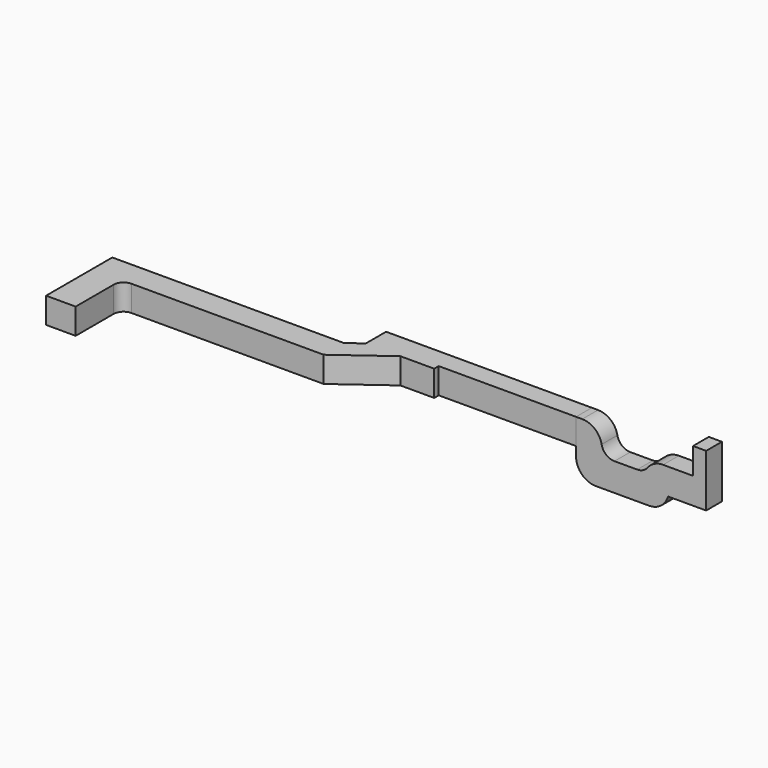
from build123d import *

# Parameters (mm, degrees)
F0_W        = 4.5
F0_H        = 8.74
F0_W_2      = 20.9
F0_H_2      = 3
F1_DEPTH    = 3.92
F0_W_3      = 19.8
F2_DEPTH    = 8.3
F3_DEPTH    = 1.88
F4_W        = 5.8
F4_H        = 2.18
F5_DEPTH    = 25
F6_T1_DEPTH = 18
F6_T3_DEPTH = 17.4287906631
F6_T5_DEPTH = 16.9987425023
F7_R        = 2
F8_R        = 1.5


# Not quite as in the source:
# - a fillet or chamfer that OpenCascade refuses, or shapes differently, is made with other operations: its cross-section is extruded or revolved along the edge and cut away or added
# - a feature names something its author has since deleted; it is built from what else it names


with BuildPart() as f1:
    # F0 (on Top) → F1 (new body)
    with BuildSketch(Plane.XY):
        with Locations((2.25, 4.37)):
            Rectangle(F0_W, F0_H)
        Polygon((0, 12.6), (0, 8.74), (4.5, 8.74), (35.25, 8.74), (35.25, 12.6), align=None)
        Polygon((35.25, 12.6), (35.25, 8.74), (42.6136363636, 14.14), (37.35, 14.14), align=None)
        Polygon((37.35, 14.14), (42.6136363636, 14.14), (47.76, 14.14), (47.76, 15), (47.76, 18), (37.35, 18), align=None)
        with Locations((58.21, 16.5)):
            Rectangle(F0_W_2, F0_H_2)
    extrude(amount=-F1_DEPTH)

    # F8
    f8_edges = [f1.edges().sort_by_distance(p)[0] for p in [
        (4.5, 8.74, -1.96),
    ]]
    fillet(f8_edges, radius=F8_R)


with BuildPart() as f2:
    # F0 (on Top) → F2 (new body)
    with BuildSketch(Plane.XY):
        with Locations((78.56, 16.5)):
            Rectangle(F0_W_3, F0_H_2)
    extrude(amount=-F2_DEPTH)

    # F0 (on Top) → F3 (join)
    with BuildSketch(Plane.XY):
        with Locations((78.56, 16.5)):
            Rectangle(F0_W_3, F0_H_2)
    extrude(amount=F3_DEPTH)

    # F4 (on face) → F5 (cut)
    with BuildSketch(Plane(origin=(0, 18, 0), x_dir=(-1, 0, 0), z_dir=(0, 1, 0))):
        with Locations((-85.56, -7.21)):
            Rectangle(F4_W, F4_H)
        Polygon((-68.66, 1.88), (-86.46, 1.88), (-86.46, -2.12), (-82.66, -2.12), (-79.1077613831, -2.12), (-79.1077613831, -4.0423134342), (-72.6052895188, -4.0423134342), (-72.6052895188, 0), (-68.66, 0), align=None)
    extrude(amount=-F5_DEPTH, mode=Mode.SUBTRACT)

    # F6: fillet of radius 3 on 4 edges, made by hand

    # F6_s2 → F6_t1 (cut)
    with BuildSketch(Plane.XZ.offset(-25.5)):
        with BuildLine():
            ThreePointArc((68.66, -5.3), (69.5386796564, -7.4213203436), (71.66, -8.3))
            Line((71.66, -8.3), (68.66, -8.3))
            Line((68.66, -8.3), (68.66, -5.3))
        make_face()
        with BuildLine():
            ThreePointArc((69.6052895188, 0), (71.7266098624, -0.8786796564), (72.6052895188, -3))
            Line((72.6052895188, -3), (72.6052895188, 0))
            Line((72.6052895188, 0), (69.6052895188, 0))
        make_face()
    extrude(amount=F6_T1_DEPTH, mode=Mode.SUBTRACT)

    # F6_s4 → F6_t3 (cut)
    with BuildSketch(Plane.XZ.offset(-25.2143953316)):
        with BuildLine():
            ThreePointArc((79.7742418674, -8.3), (81.5825559994, -7.6937418407), (82.66, -6.12))
            Line((82.66, -6.12), (82.66, -8.3))
            Line((82.66, -8.3), (79.7742418674, -8.3))
        make_face()
    extrude(amount=F6_T3_DEPTH, mode=Mode.SUBTRACT)

    # F6_s6 → F6_t5 (cut)
    with BuildSketch(Plane.XZ.offset(-24.9993712512)):
        with BuildLine():
            ThreePointArc((81.9075098835, -2.12), (80.2094315133, -2.6468380868), (79.1077613831, -4.0423134342))
            Line((79.1077613831, -4.0423134342), (79.1077613831, -2.12))
            Line((79.1077613831, -2.12), (81.9075098835, -2.12))
        make_face()
    extrude(amount=F6_T5_DEPTH, mode=Mode.SUBTRACT)

    # F7
    f7_edges = [f2.edges().sort_by_distance(p)[0] for p in [
        (72.60529, 16.5, -4.042313),
        (79.107761, 16.5, -4.042313),
    ]]
    fillet(f7_edges, radius=F7_R)


solid = Compound([f1.part, f2.part])
